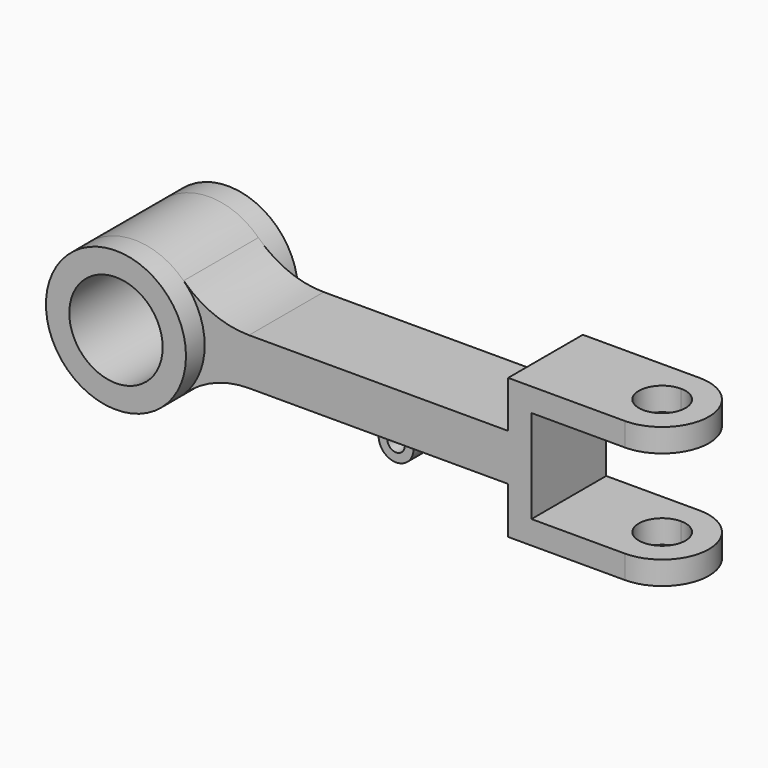
from build123d import *

# Parameters (mm, degrees)
F0_R        = 25.4
F1_DEPTH    = 50.8
F2_R        = 38.1
F2_R_2      = 25.4
F3_DEPTH    = 12.7
F4_R        = 38.1
F4_R_2      = 25.4
F5_DEPTH    = 12.7
F6_T1_DEPTH = 50.8
F7_R        = 12.7
F8_DEPTH    = 12.7
F10_DEPTH   = 12.7
F11_DEPTH   = 76.201
F14_DEPTH   = 6.35


# Not quite as in the source:
# - a fillet or chamfer that OpenCascade refuses, or shapes differently, is made with other operations: its cross-section is extruded or revolved along the edge and cut away or added
# - a feature names something its author has since deleted; it is built from what else it names


with BuildPart() as f1:
    # F0 (on Front) → F1 (new body)
    with BuildSketch(Plane.XZ):
        with BuildLine():
            ThreePointArc((35.921024, -12.7), (37.551305, -6.442785), (38.1, 0))
            ThreePointArc((38.1, 0), (37.551305, 6.442785), (35.921024, 12.7))
            ThreePointArc((35.921024, 12.7), (-38.1, 0), (35.921024, -12.7))
        make_face()
        Circle(F0_R, mode=Mode.SUBTRACT)
        with BuildLine():
            ThreePointArc((35.921024, 12.7), (37.551305, 6.442785), (38.1, 0))
            ThreePointArc((38.1, 0), (37.551305, -6.442785), (35.921024, -12.7))
            Line((35.921024, -12.7), (203.2, -12.7))
            Line((203.2, -12.7), (203.2, 0))
            Line((203.2, 0), (203.2, 12.7))
            Line((203.2, 12.7), (35.921024, 12.7))
        make_face()
        Polygon((203.2, 38.1), (203.2, 12.7), (203.2, 0), (203.2, -12.7), (203.2, -38.1), (266.7, -38.1), (266.7, -25.4), (215.9, -25.4), (215.9, 25.4), (266.7, 25.4), (266.7, 38.1), align=None)
    extrude(amount=F1_DEPTH)

    # F2 (on face) → F3 (join)
    with BuildSketch(Plane.XZ.offset(50.8)):
        Circle(F2_R)
        Circle(F2_R_2, mode=Mode.SUBTRACT)
    extrude(amount=F3_DEPTH)

    # F4 (on face) → F5 (join)
    with BuildSketch(Plane(origin=(0, 0, 0), x_dir=(-1, 0, 0), z_dir=(0, 1, 0))):
        Circle(F4_R)
        Circle(F4_R_2, mode=Mode.SUBTRACT)
    extrude(amount=F5_DEPTH)

    # F6: fillet of radius 50.8 on 2 edges, made by hand

    # F6_s2 → F6_t1 (join)
    with BuildSketch(Plane.XZ):
        with BuildLine():
            ThreePointArc((26.664445, -27.214286), (43.016444, -16.468339), (62.217039, -12.7))
            Line((62.217039, -12.7), (35.921024, -12.7))
            ThreePointArc((35.921024, -12.7), (32.123222, -20.486791), (26.664445, -27.214286))
        make_face()
        with BuildLine():
            ThreePointArc((62.217039, 12.7), (43.016444, 16.468339), (26.664445, 27.214286))
            ThreePointArc((26.664445, 27.214286), (32.123222, 20.486791), (35.921024, 12.7))
            Line((35.921024, 12.7), (62.217039, 12.7))
        make_face()
    extrude(amount=F6_T1_DEPTH)

    # F7 (on face) → F8 (join)
    with BuildSketch(Plane(origin=(0, 0, -38.1), x_dir=(1, 0, 0), z_dir=(0, 0, -1))):
        with Locations((266.7, 25.4)):
            Circle(F7_R)
        with BuildLine():
            Line((266.7, 12.7), (266.7, 0))
            ThreePointArc((266.7, 0), (292.1, 25.4), (266.7, 50.8))
            Line((266.7, 50.8), (266.7, 38.1))
            ThreePointArc((266.7, 38.1), (275.680256, 34.380256), (279.4, 25.4))
            ThreePointArc((279.4, 25.4), (275.680256, 16.419744), (266.7, 12.7))
        make_face()
    extrude(amount=-F8_DEPTH)

    # F9 (on face) → F10 (join)
    with BuildSketch(Plane.XY.offset(38.1)):
        with BuildLine():
            Line((266.7, 0), (266.7, -50.8))
            ThreePointArc((266.7, -50.8), (292.1, -25.4), (266.7, 0))
        make_face()
    extrude(amount=-F10_DEPTH)

    # F7 (on face) → F11 (cut, through all)
    with BuildSketch(Plane(origin=(0, 0, -38.1), x_dir=(1, 0, 0), z_dir=(0, 0, -1))):
        with BuildLine():
            Line((266.7, 38.1), (266.7, 12.7))
            ThreePointArc((266.7, 12.7), (275.680256, 16.419744), (279.4, 25.4))
            ThreePointArc((279.4, 25.4), (275.680256, 34.380256), (266.7, 38.1))
        make_face()
        with BuildLine():
            ThreePointArc((266.7, 38.1), (254, 25.4), (266.7, 12.7))
            Line((266.7, 12.7), (266.7, 38.1))
        make_face()
    extrude(amount=-F11_DEPTH, mode=Mode.SUBTRACT)

    # F13 (on offset) → F14 (join, symmetric)
    with BuildSketch(Plane(origin=(0, -25.4, 0), x_dir=(-1, 0, 0), z_dir=(0, 1, 0))):
        with BuildLine():
            Line((-117.475, -25.4), (-117.475, -12.7))
            Line((-117.475, -12.7), (-136.525, -12.7))
            Line((-136.525, -12.7), (-136.525, -25.4))
            Line((-136.525, -25.4), (-131.7625, -25.4))
            ThreePointArc((-131.7625, -25.4), (-127, -20.6375), (-122.2375, -25.4))
            Line((-122.2375, -25.4), (-117.475, -25.4))
        make_face()
        with BuildLine():
            ThreePointArc((-136.525, -25.4), (-127, -34.925), (-117.475, -25.4))
            Line((-117.475, -25.4), (-122.2375, -25.4))
            ThreePointArc((-122.2375, -25.4), (-127, -30.1625), (-131.7625, -25.4))
            Line((-131.7625, -25.4), (-136.525, -25.4))
        make_face()
    extrude(amount=F14_DEPTH, both=True)


solid = f1.part
